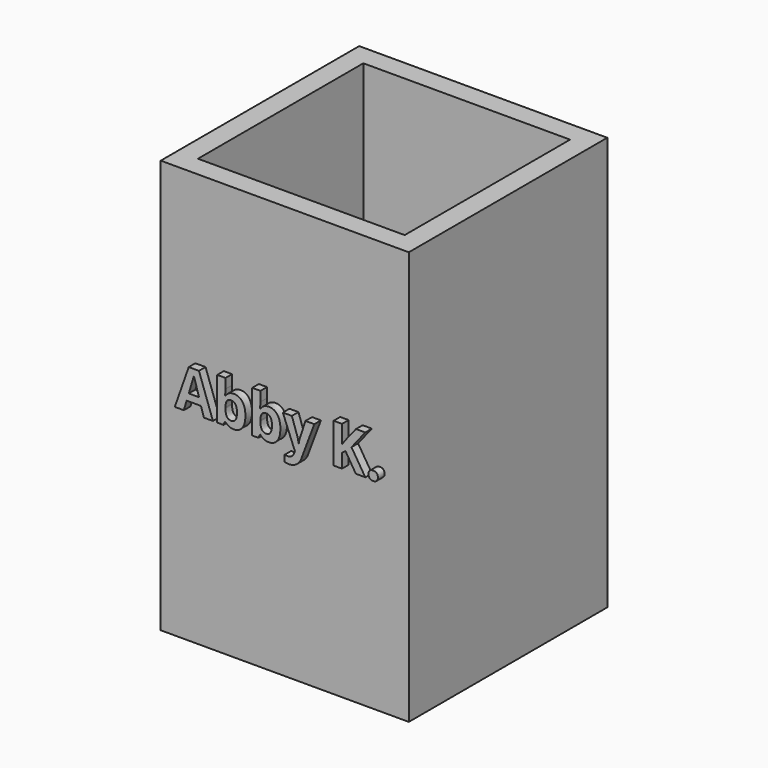
from build123d import *

# Parameters (mm, degrees)
F0_W         = 76.2
F0_H         = 127
F1_DEPTH     = 76.2
F2_W         = 63.5
F2_H         = 63.5
F3_DEPTH     = 120.65
F4_TEXT_SIZE = 16.9729368527
F5_DEPTH     = 2.54


# Not quite as in the source:
# - Text() gives the source's letters only with a copy of the font that has no kerning and outlines rounded to 1/6400 em; it was checked with that copy


with BuildPart() as f1:
    # F0 (on Front) → F1 (new body)
    with BuildSketch(Plane.XZ):
        with Locations((10.6295013472, 25.4193049216)):
            Rectangle(F0_W, F0_H)
    extrude(amount=F1_DEPTH)

    # F2 (on face) → F3 (cut)
    with BuildSketch(Plane.XY.offset(88.9193049216)):
        with Locations((10.6295013472, -38.1)):
            Rectangle(F2_W, F2_H)
    extrude(amount=-F3_DEPTH, mode=Mode.SUBTRACT)

    # F4 (on face) → F5 (join)
    with BuildSketch(Plane.XZ.offset(76.2)):
        with Locations((-21.1204986528, 25.4193049216)):
            Text('Abby K.', F4_TEXT_SIZE, font='Open Sans', font_style=FontStyle.BOLD, text_align=(TextAlign.LEFT, TextAlign.BOTTOM))
    extrude(amount=F5_DEPTH)


solid = f1.part
